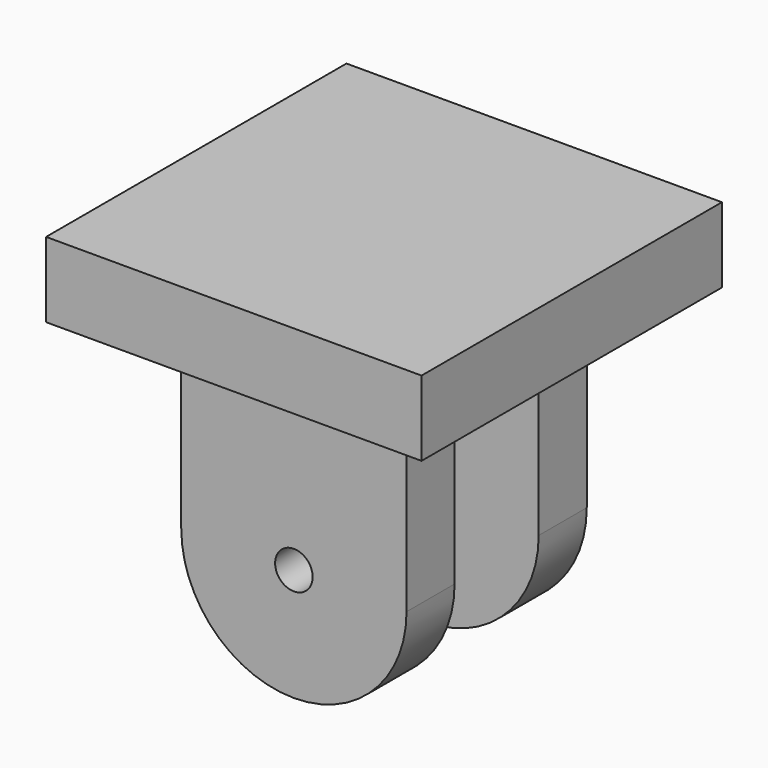
from build123d import *

# Parameters (mm, degrees)
F0_W     = 50
F0_H     = 50
F1_DEPTH = 10
F3_DEPTH = 40
F4_R     = 15
F5_R     = 15
F6_R     = 14.99999
F7_R     = 14.99999
F9_D     = 5


# Not quite as in the source:
# - a fillet or chamfer is up to 0.001 mm smaller than in the source, because OpenCascade refuses the exact size


with BuildPart() as f1:
    # F0 (on Top) → F1 (new body)
    with BuildSketch(Plane.XY):
        with Locations((2.4681314826, -1.799523242)):
            Rectangle(F0_W, F0_H)
    extrude(amount=F1_DEPTH)

    # F2 (on face) → F3 (join)
    with BuildSketch(Plane(origin=(0, 0, 0), x_dir=(1, 0, 0), z_dir=(0, 0, -1))):
        Polygon((2.4681314826, 16.799523242), (-12.5318685174, 16.799523242), (-12.5318685174, 8.799523242), (17.4681314826, 8.799523242), (17.4681314826, 12.799523242), (17.4681314826, 16.799523242), align=None)
        Polygon((-12.5318685174, -5.200476758), (-12.5318685174, -9.200476758), (-12.5318685174, -13.200476758), (2.4681314826, -13.200476758), (17.4681314826, -13.200476758), (17.4681314826, -5.200476758), align=None)
    extrude(amount=F3_DEPTH)

    # F4
    f4_edges = [f1.edges().sort_by_distance(p)[0] for p in [
        (17.468131, 9.200477, -40),
    ]]
    fillet(f4_edges, radius=F4_R)

    # F5
    f5_edges = [f1.edges().sort_by_distance(p)[0] for p in [
        (17.468131, -12.799523, -40),
    ]]
    fillet(f5_edges, radius=F5_R)

    # F6 (radius 15 in the source; OpenCascade refuses exactly that, so slightly less here)
    f6_edges = [f1.edges().sort_by_distance(p)[0] for p in [
        (-12.531869, 9.200477, -40),
    ]]
    fillet(f6_edges, radius=F6_R)

    # F7 (radius 15 in the source; OpenCascade refuses exactly that, so slightly less here)
    f7_edges = [f1.edges().sort_by_distance(p)[0] for p in [
        (-12.531869, -12.799523, -40),
    ]]
    fillet(f7_edges, radius=F7_R)

    # F9 (through all)
    with Locations(Plane(origin=(0, 13.200476758, 0), x_dir=(-1, 0, 0), z_dir=(0, 1, 0))):
        with Locations((-2.4681314826, -25)):
            Hole(F9_D / 2)


solid = f1.part
